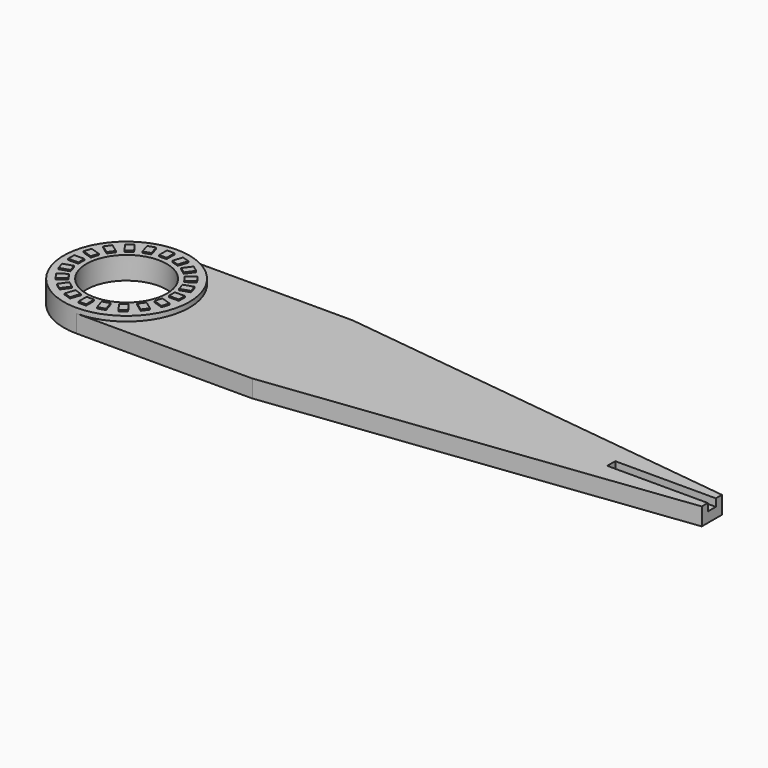
from build123d import *

# Parameters (mm, degrees)
F0_R         = 8
F1_DEPTH     = 3.5
F2_R         = 12.5
F2_R_2       = 8
F3_DEPTH     = 1
F4_W         = 1.5
F4_H         = 2
F4_W_2       = 2
F4_H_2       = 1.5
F5_DEPTH     = 0.25
F6_W         = 20
F6_H         = 2
F7_DEPTH     = 1.5
F8_TEXT_SIZE = 16.6742292802
F9_DEPTH     = 1


# Not quite as in the source:
# - Text() gives the source's letters only with a copy of the font that has no kerning and outlines rounded to 1/6400 em; it was checked with that copy


with BuildPart() as f1:
    # F0 (on Top) → F1 (new body)
    with BuildSketch(Plane.XY):
        with BuildLine():
            ThreePointArc((0, -12.5), (8.8388347648, -8.8388347648), (12.5, 0))
            ThreePointArc((12.5, 0), (8.8388347648, 8.8388347648), (0, 12.5))
            ThreePointArc((0, 12.5), (-12.5, 0), (0, -12.5))
        make_face()
        Circle(F0_R, mode=Mode.SUBTRACT)
        with BuildLine():
            ThreePointArc((0, 12.5), (8.8388347648, 8.8388347648), (12.5, 0))
            ThreePointArc((12.5, 0), (8.8388347648, -8.8388347648), (0, -12.5))
            Line((0, -12.5), (35, -12.5))
            Line((35, -12.5), (116.3887844346, -2.5067138408))
            Line((116.3887844346, -2.5067138408), (116.3887844346, 2.5067138408))
            Line((116.3887844346, 2.5067138408), (35, 12.5))
            Line((35, 12.5), (0, 12.5))
        make_face()
    extrude(amount=F1_DEPTH)

    # F2 (on face) → F3 (join)
    with BuildSketch(Plane.XY.offset(3.5)):
        Circle(F2_R)
        Circle(F2_R_2, mode=Mode.SUBTRACT)
    extrude(amount=F3_DEPTH)

    # F4 (on face) → F5 (join)
    with BuildSketch(Plane.XY.offset(4.5)):
        with Locations((0, 10)):
            Rectangle(F4_W, F4_H)
        Polygon((-2.6858945509, 10.693384425), (-4.1124793253, 10.2298589335), (-3.4944453366, 8.3277459009), (-2.0678605622, 8.7912713924), align=None)
        Polygon((-5.8588750294, 9.3400258773), (-7.072400521, 8.4583479989), (-5.8968300164, 6.8403140102), (-4.6833045249, 7.7219918886), align=None)
        Polygon((-8.4583479989, 7.072400521), (-9.3400258773, 5.8588750294), (-7.7219918886, 4.6833045249), (-6.8403140102, 5.8968300164), align=None)
        Polygon((-10.2298589335, 4.1124793253), (-10.693384425, 2.6858945509), (-8.7912713924, 2.0678605622), (-8.3277459009, 3.4944453366), align=None)
        with Locations((-10, 0)):
            Rectangle(F4_W_2, F4_H_2)
        Polygon((-10.693384425, -2.6858945509), (-10.2298589335, -4.1124793253), (-8.3277459009, -3.4944453366), (-8.7912713924, -2.0678605622), align=None)
        Polygon((-9.3400258773, -5.8588750294), (-8.4583479989, -7.072400521), (-6.8403140102, -5.8968300164), (-7.7219918886, -4.6833045249), align=None)
        Polygon((-7.072400521, -8.4583479989), (-5.8588750294, -9.3400258773), (-4.6833045249, -7.7219918886), (-5.8968300164, -6.8403140102), align=None)
        Polygon((-4.1124793253, -10.2298589335), (-2.6858945509, -10.693384425), (-2.0678605622, -8.7912713924), (-3.4944453366, -8.3277459009), align=None)
        with Locations((0, -10)):
            Rectangle(F4_W, F4_H)
        Polygon((2.6858945509, -10.693384425), (4.1124793253, -10.2298589335), (3.4944453366, -8.3277459009), (2.0678605622, -8.7912713924), align=None)
        Polygon((5.8588750294, -9.3400258773), (7.072400521, -8.4583479989), (5.8968300164, -6.8403140102), (4.6833045249, -7.7219918886), align=None)
        Polygon((8.4583479989, -7.072400521), (9.3400258773, -5.8588750294), (7.7219918886, -4.6833045249), (6.8403140102, -5.8968300164), align=None)
        Polygon((10.2298589335, -4.1124793253), (10.693384425, -2.6858945509), (8.7912713924, -2.0678605622), (8.3277459009, -3.4944453366), align=None)
        with Locations((10, 0)):
            Rectangle(F4_W_2, F4_H_2)
        Polygon((10.693384425, 2.6858945509), (10.2298589335, 4.1124793253), (8.3277459009, 3.4944453366), (8.7912713924, 2.0678605622), align=None)
        Polygon((9.3400258773, 5.8588750294), (8.4583479989, 7.072400521), (6.8403140102, 5.8968300164), (7.7219918886, 4.6833045249), align=None)
        Polygon((7.072400521, 8.4583479989), (5.8588750294, 9.3400258773), (4.6833045249, 7.7219918886), (5.8968300164, 6.8403140102), align=None)
        Polygon((4.1124793253, 10.2298589335), (2.6858945509, 10.693384425), (2.0678605622, 8.7912713924), (3.4944453366, 8.3277459009), align=None)
    extrude(amount=F5_DEPTH)

    # F6 (on face) → F7 (cut)
    with BuildSketch(Plane.XY.offset(3.5)):
        with Locations((106.3887844346, -0.0067138408)):
            Rectangle(F6_W, F6_H)
    extrude(amount=-F7_DEPTH, mode=Mode.SUBTRACT)

    # F8 (on face) → F9 (cut)
    with BuildSketch(Plane(origin=(0, 0, 0), x_dir=(1, 0, 0), z_dir=(0, 0, -1))):
        with Locations((15.8350411803, -6.4314887859)):
            Text('Fish', F8_TEXT_SIZE, font='Open Sans', text_align=(TextAlign.LEFT, TextAlign.BOTTOM))
    extrude(amount=-F9_DEPTH, mode=Mode.SUBTRACT)


solid = f1.part
